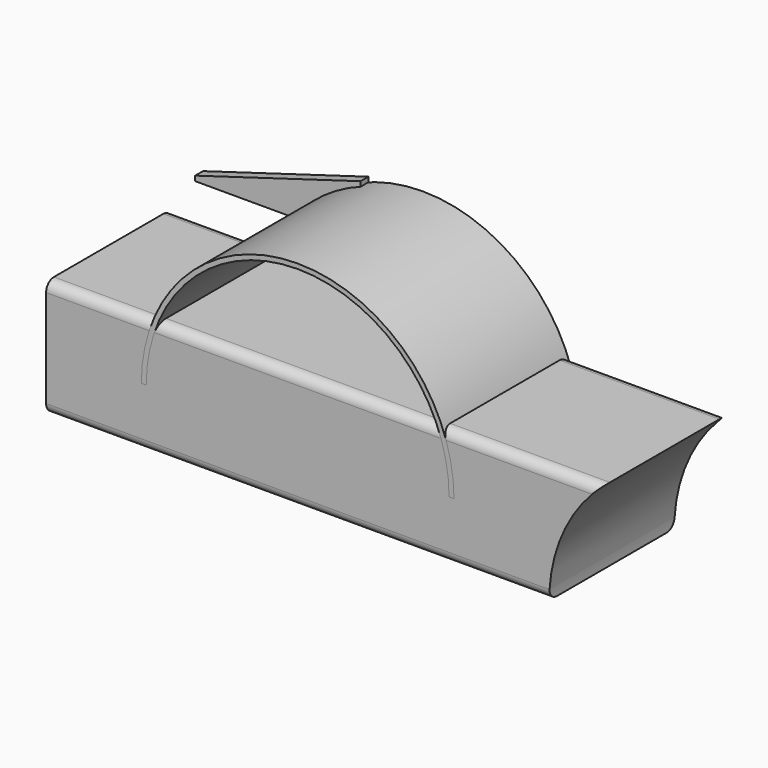
from build123d import *

# Parameters (mm, degrees)
F1_DEPTH = 101.6
F2_R     = 6.35
F3_T     = 6.35
F5_DEPTH = 101.6
F7_DEPTH = 6.35


# Not quite as in the source:
# - a shell that OpenCascade refuses in one call is made with other operations: the cavity is built on its own and cut out


with BuildPart() as f1:
    # F0 (on Front) → F1 (new body)
    with BuildSketch(Plane.XZ):
        with BuildLine():
            Line((197.910416699, 38.1), (163.5125, 38.1))
            Line((163.5125, 38.1), (-163.5125, 38.1))
            Line((-163.5125, 38.1), (-163.5125, -38.1))
            Line((-163.5125, -38.1), (163.5125, -38.1))
            ThreePointArc((163.5125, -38.1), (172.510416699, 3.702083301), (197.910416699, 38.1))
        make_face()
    extrude(amount=F1_DEPTH)

    # F2
    f2_edges = [f1.edges().sort_by_distance(p)[0] for p in [
        (17.198958, -101.6, 38.1),
        (0, -101.6, -38.1),
        (17.198958, 0, 38.1),
        (0, 0, -38.1),
    ]]
    fillet(f2_edges, radius=F2_R)

    # F3: shell of thickness 6.35, made by hand


with BuildPart() as f3_core1:
    # F3_t2: copy of F1
    add(f1.part)

    # the walls: a layer under each face that stays
    f3_faces = [f3_core1.faces().sort_by_distance(p)[0] for p in [
        (172.510416699, -50.8, 3.702083301),
        (0, -50.8, -38.1),
        (13.9098336274, 0, 0),
        (13.9098336274, -101.6, 0),
        (17.1989583495, -50.8, 38.1),
    ]]
    thicken(f3_faces, amount=-F3_T, mode=Mode.SUBTRACT)


with BuildPart() as f1_1:
    add(f1.part)

    # what is left inside the walls is the cavity
    f3_cavity = [f3_core1.part.solids().sort_by_distance(p)[0] for p in [
        (9.647297, -65.616667, 31.6865),
    ]]
    add(f3_cavity, mode=Mode.SUBTRACT)


with BuildPart() as f5:
    # F4 (on Front) → F5 (new body)
    with BuildSketch(Plane.XZ):
        with BuildLine():
            Line((98.425, 0), (101.6, 0))
            ThreePointArc((101.6, 0), (0, 101.6), (-101.6, 0))
            Line((-101.6, 0), (-98.425, 0))
            ThreePointArc((-98.425, 0), (0, 98.425), (98.425, 0))
        make_face()
    extrude(amount=F5_DEPTH)


with BuildPart() as f7:
    # F6 (on Front) → F7 (new body)
    with BuildSketch(Plane.XZ):
        with BuildLine():
            ThreePointArc((-79.3114745797, 63.5), (-59.4906138436, 82.3615618144), (-35.355303704, 95.25))
            Line((-35.355303704, 95.25), (-35.355303704, 98.425))
            Line((-35.355303704, 98.425), (-142.8114745797, 66.675))
            Line((-142.8114745797, 66.675), (-142.8114745797, 63.5))
            Line((-142.8114745797, 63.5), (-79.3114745797, 63.5))
        make_face()
    extrude(amount=F7_DEPTH)


solid = Compound([f1_1.part, f5.part, f7.part])
